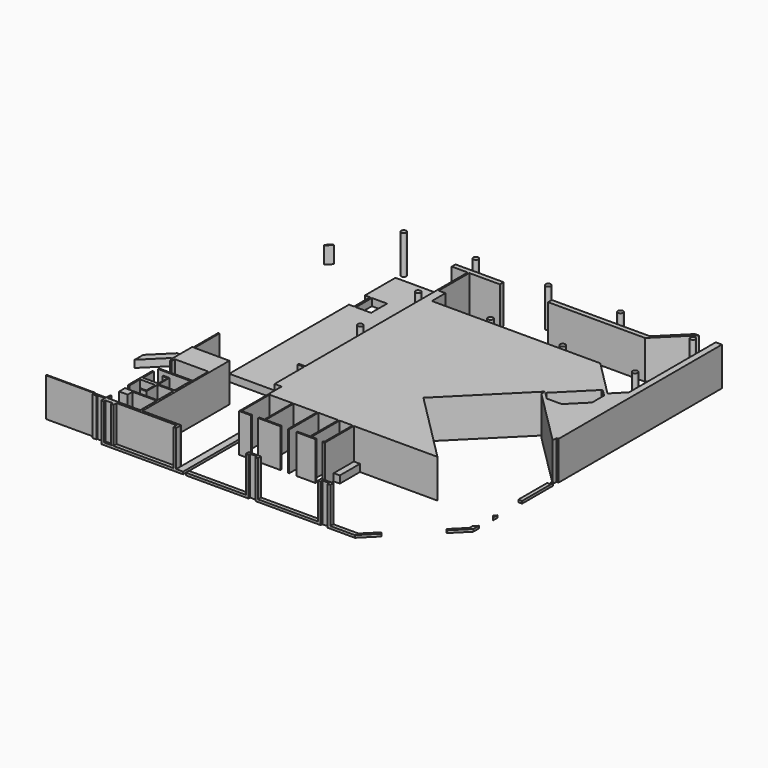
from build123d import *

# Parameters (mm, degrees)
F0_W      = 988.1219863892
F0_H      = 168.411863653
F1_DEPTH  = 4876.8
F0_R      = 328.452152689
F0_W_2    = 6102.4697852615
F0_H_2    = 118.2537078857
F2_DEPTH  = 914.4
F0_W_3    = 1924.9444007874
F0_H_3    = 2527.5359153748
F0_W_4    = 159.9474188251
F0_H_4    = 572.0329284668
F0_W_5    = 776.8564224243
F0_H_5    = 3188.3936524391
F3_DEPTH  = 177.8
F4_DEPTH  = 355.6
F5_DEPTH  = 533.4
F6_DEPTH  = 711.2
F7_DEPTH  = 889
F8_DEPTH  = 1066.8
F9_DEPTH  = 2133.6
F0_W_6    = 878.3769310551
F0_H_6    = 490.4985427856
F0_H_7    = 289.0536963655
F0_H_8    = 17331.1824798584
F0_H_9    = 184.3700408936
F0_H_10   = 7452.3627518665
F10_DEPTH = 304.8
F0_W_7    = 7604.6065750122
F0_W_8    = 7599.9544025821
F0_W_9    = 331.0794830322
F11_DEPTH = 4876.8


with BuildPart() as f1:
    # F0 (on Top) → F1 (new body)
    with BuildSketch(Plane.XY):
        Polygon((-9762.6952889996, -31763.6391877186), (-9950.2172235089, -31763.6391877186), (-9950.2172235089, -32382.503724004), (-9950.2172235089, -32550.915587657), (-9950.2172235089, -33159.8601280416), (-9619.1377404767, -33159.8601280416), (-9619.1377404767, -32907.453054067), (-8738.1992105084, -32907.453054067), (-8738.1992105084, -33145.5445228781), (-8410.8237985211, -33145.5445228781), (-8410.8237985211, -32669.361585256), (-806.2172235089, -32669.361585256), (-475.1377404767, -32669.361585256), (-475.1377404767, -32380.3078888905), (-5368.5698274213, -32380.3078888905), (-5368.5698274213, -18630.5877923023), (-9778.8629296857, -18630.5877923023), (-9778.8629296857, -15049.1254090321), (-9778.8629296857, -14864.7553681385), (-9778.8629296857, -14666.6457413685), (-9938.8103485107, -14666.6457413685), (-9938.8103485107, -15837.9578638238), (-9938.8103485107, -18630.5877923023), (-10073.0752944946, -18630.5877923023), (-10073.0752944946, -21932.6489324318), (-9941.6446450787, -21932.6489324318), (-9941.9820483797, -22319.5813578577), (-9762.6952889996, -22319.7376950899), (-9762.6952889996, -21738.5065316212), (-5534.9635842877, -21738.5065316212), (-5534.9635842877, -24228.4532546055), (-9762.6952889996, -24255.6560992252), (-9762.6952889996, -24422.071790601), (-5641.0493615704, -24422.071790601), (-5641.0493615704, -26945.4772233021), (-7697.0572236615, -26945.4772233021), (-7697.0572236615, -25199.2787479412), (-8474.8048782349, -25199.2787479412), (-8474.8048782349, -25341.5817229998), (-7804.6655419904, -25341.5817229998), (-7804.6655419904, -26805.3394316685), (-9762.6952889996, -26805.3394316685), (-9762.6952889996, -25341.5817229998), (-9762.6952889996, -25199.2787479412), (-9762.6952889996, -25087.7745624565), (-9944.395762002, -25087.6161204771), (-9947.7741608292, -28961.9470722609), (-9762.6952889996, -28961.9470722609), (-9762.6952889996, -28854.1154622089), (-9762.6952889996, -28712.3789547932), (-9762.6952889996, -27257.7159165394), (-7818.7813523846, -27257.7159165394), (-7818.7813523846, -28712.3789547932), (-8473.2656478882, -28712.3789547932), (-8473.2656478882, -28854.1154622089), (-7684.504962309, -28854.1154622089), (-7697.0572236615, -27101.0598896992), (-6705.3122520447, -27101.0598896992), (-5641.0493615704, -27101.0598896992), (-5641.0493615704, -27707.3329574996), (-5641.0493615704, -29643.5177086842), (-9762.6952889996, -29643.5177086842), (-9762.6952889996, -30572.3111390125), (-8683.9914086896, -30572.3111390125), (-8683.9914086896, -29799.5407341969), (-5641.0493615704, -29799.5407341969), (-5641.0493615704, -32380.3078888905), (-9762.6952889996, -32380.3078888905), align=None)
        Polygon((-10938.3392098981, -32550.915587657), (-10938.3392098981, -32382.503724004), (-11455.8429483014, -32382.503724004), (-11455.8429483014, -32680.3834198963), (-10938.3392098981, -32680.3834198963), align=None)
        with Locations((-10444.2782167035, -32466.7096558305)):
            Rectangle(F0_W, F0_H)
    extrude(amount=F1_DEPTH)

    # F0 (on Top) → F10 (join)
    with BuildSketch(Plane.XY):
        Polygon((-9619.1377404767, -32907.453054067), (-9619.1377404767, -33159.8601280416), (-806.2172235089, -33159.8601280416), (-806.2172235089, -32669.361585256), (-8410.8237985211, -32669.361585256), (-8410.8237985211, -33145.5445228781), (-8738.1992105084, -33145.5445228781), (-8738.1992105084, -32907.453054067), align=None)
        with Locations((-35.9492749491, -32914.6108566488)):
            Rectangle(F0_W_6, F0_H_6)
        with Locations((-35.9492749491, -32524.8347370732)):
            Rectangle(F0_W_6, F0_H_7)
        with Locations((-35.9492749491, -23714.7166489613)):
            Rectangle(F0_W_6, F0_H_8)
        with Locations((-35.9492749491, -14956.9403885853)):
            Rectangle(F0_W_6, F0_H_9)
        with Locations((-35.9492749491, -11138.5739922052)):
            Rectangle(F0_W_6, F0_H_10)
    extrude(amount=F10_DEPTH)


with BuildPart() as f1b:
    # F0 (on Top) → F1, piece 2 (new body)
    with BuildSketch(Plane.XY):
        Polygon((403.2391905785, -14864.7553681385), (403.2391905785, -15049.1254090321), (1221.1445804996, -15049.1254090321), (1221.1445804996, -19710.1065873158), (2114.7113081378, -19710.1065873158), (2114.7113081378, -20655.0921089583), (2114.7113081378, -20733.6380242359), (2114.7113081378, -26433.5496782314), (3611.5431785584, -26433.5496782314), (3611.5431785584, -26267.01645922), (2270.482301712, -26267.01645922), (2270.482301712, -21826.6788608962), (5186.9406700134, -21826.6788608962), (5186.9406700134, -26267.01645922), (4527.3551940918, -26267.01645922), (4527.3551940918, -26433.5496782314), (7342.5350189209, -26433.5496782314), (7342.5350189209, -26267.01645922), (5332.866191864, -26267.01645922), (5332.866191864, -21826.6788608962), (8282.6271057129, -21826.6788608962), (8282.6271057129, -26267.01645922), (8282.6271057129, -26433.5496782314), (8448.1201171875, -26433.5496782314), (8448.1201171875, -26267.01645922), (8448.1201171875, -21826.6788608962), (10967.3471450806, -21826.6788608962), (10967.3471450806, -26267.01645922), (9387.3443603516, -26267.01645922), (9387.3443603516, -26433.5496782314), (11770.4105377197, -26433.5496782314), (11770.4105377197, -26267.01645922), (11142.1804428101, -26267.01645922), (11142.1804428101, -21826.6788608962), (12795.4187393188, -21826.6788608962), (12795.4187393188, -26267.01645922), (12655.650138855, -26267.01645922), (12655.650138855, -26433.5496782314), (12953.9604422015, -26433.5496782314), (12953.9604422015, -25034.6246122372), (12953.9604422015, -21846.2309597981), (13730.8168646259, -21846.2309597981), (23534.5983740253, -21846.2309597981), (14549.2862374604, -12835.417128042), (23102.8533115337, -4306.0576854206), (23102.8533115337, -4877.016544342), (30215.8937689227, -11970.8853073243), (30215.8937689227, -11358.6764274801), (30472.748779909, -11358.6764274801), (30472.748779909, 14474.1640090942), (29691.0285949707, 14474.1640090942), (29691.0285949707, 751.9209384918), (28176.9048769071, -757.9176259485), (27421.1322496944, 0), (23591.3720324397, 3840.629664663), (2272.8099822998, 3840.629664663), (2272.8099822998, 5998.2261657715), (1416.9044729633, 5998.2261657715), (1416.9044729633, 10830.4662704468), (1221.1445804996, 10830.4662704468), (1221.1445804996, -14864.7553681385), align=None)
        with Locations((9121.6776853174, -4581.9952062592)):
            Circle(F0_R, mode=Mode.SUBTRACT)
        with Locations((18270.2025953174, -4581.9952062592)):
            Circle(F0_R, mode=Mode.SUBTRACT)
        Polygon((23372.4136352539, -4562.3035430908), (23372.4136352539, -4424.2610931396), (27250.2002716064, -545.2130857547), (27426.9443765413, -545.2130857547), (28200.6041700507, -1321.0686445236), (28200.6041700507, -2802.8049468994), (28200.6041700507, -3235.0963548069), (26065.6871795654, -5363.9712714722), (24176.2479287661, -5363.9712714722), align=None, mode=Mode.SUBTRACT)
        with Locations((9121.6776853174, -4581.9952062592)):
            Circle(F0_R)
        with Locations((18270.2025953174, -4581.9952062592)):
            Circle(F0_R)
        Polygon((-798.6393335896, 11424.7198104858), (-798.6393335896, 10830.4662704468), (1221.1445804996, 10830.4662704468), (1416.9044729633, 10830.4662704468), (5292.9373022479, 10830.4662704468), (5292.9373022479, 11424.7198104858), align=None)
    extrude(amount=F1_DEPTH)


with BuildPart() as f1c:
    # F0 (on Top) → F1, piece 3 (new body)
    with BuildSketch(Plane.XY):
        with Locations((-26.8472246826, 4554.5749137408)):
            Circle(F0_R)
    extrude(amount=F1_DEPTH)


with BuildPart() as f1d:
    # F0 (on Top) → F1, piece 4 (new body)
    with BuildSketch(Plane.XY):
        with Locations((-26.8472246826, -4581.9952062592)):
            Circle(F0_R)
    extrude(amount=F1_DEPTH)


with BuildPart() as f1e:
    # F0 (on Top) → F1, piece 5 (new body)
    with BuildSketch(Plane.XY):
        with Locations((-9163.0339622498, 13691.67878642)):
            Circle(F0_R)
    extrude(amount=F1_DEPTH)


with BuildPart() as f1f:
    # F0 (on Top) → F1, piece 6 (new body)
    with BuildSketch(Plane.XY):
        with Locations((-26.8472246826, 13691.1450337408)):
            Circle(F0_R)
    extrude(amount=F1_DEPTH)


with BuildPart() as f1g:
    # F0 (on Top) → F1, piece 7 (new body)
    with BuildSketch(Plane.XY):
        with Locations((9121.6776853174, 4554.5749137408)):
            Circle(F0_R)
    extrude(amount=F1_DEPTH)


with BuildPart() as f1h:
    # F0 (on Top) → F1, piece 8 (new body)
    with BuildSketch(Plane.XY):
        with Locations((9121.6776853174, 13691.1450337408)):
            Circle(F0_R)
    extrude(amount=F1_DEPTH)


with BuildPart() as f1i:
    # F0 (on Top) → F1, piece 9 (new body)
    with BuildSketch(Plane.XY):
        with Locations((18270.2025953174, 13691.1450337408)):
            Circle(F0_R)
    extrude(amount=F1_DEPTH)


with BuildPart() as f1j:
    # F0 (on Top) → F1, piece 10 (new body)
    with BuildSketch(Plane.XY):
        with Locations((18270.2025953174, 4554.5749137408)):
            Circle(F0_R)
    extrude(amount=F1_DEPTH)


with BuildPart() as f1k:
    # F0 (on Top) → F1, piece 11 (new body)
    with BuildSketch(Plane.XY):
        with Locations((27432.5160980225, 4548.7937927246)):
            Circle(F0_R)
    extrude(amount=F1_DEPTH)


with BuildPart() as f1l:
    # F0 (on Top) → F1, piece 12 (new body)
    with BuildSketch(Plane.XY):
        with Locations((27415.8744812012, 13708.9691162109)):
            Circle(F0_R)
    extrude(amount=F1_DEPTH)


with BuildPart() as f1m:
    # F0 (on Top) → F1, piece 13 (new body)
    with BuildSketch(Plane.XY):
        with Locations((-14507.0778409321, -32323.3768700611)):
            Rectangle(F0_W_2, F0_H_2)
    extrude(amount=F1_DEPTH)


with BuildPart() as f1n:
    # F0 (on Top) → F1, piece 14 (new body)
    with BuildSketch(Plane.XY):
        Polygon((23506.2954206457, 11424.7198104858), (11396.935486452, 11424.7198104858), (11396.935486452, 10830.4662704468), (23674.6969458026, 10830.4662704468), (27462.4419350844, 14581.0467946258), (26998.763107912, 14581.0467946258), (23811.1601110858, 11424.7198104858), (23591.9761657715, 11424.7198104858), align=None)
    extrude(amount=F1_DEPTH)

    # F0 (on Top) → F3 (join)
    with BuildSketch(Plane.XY):
        Polygon((20380.9375762939, 14581.0467946258), (23506.2954206457, 11424.7198104858), (23591.9761657715, 11424.7198104858), (23773.1500730023, 11604.1160818484), (23772.2745090816, 11605.0003217233), (20825.4283058909, 14581.0467946258), align=None)
    extrude(amount=F3_DEPTH)

    # F0 (on Top) → F4 (join)
    with BuildSketch(Plane.XY):
        Polygon((21236.7263575649, 14581.0467946258), (20825.4283058909, 14581.0467946258), (23772.2745090816, 11605.0003217233), (23979.9512134187, 11810.6393509654), (23977.6984338147, 11812.91445334), align=None)
    extrude(amount=F4_DEPTH)

    # F0 (on Top) → F5 (join)
    with BuildSketch(Plane.XY):
        Polygon((21619.1883087158, 14581.0467946258), (21236.7263575649, 14581.0467946258), (23977.6984338147, 11812.91445334), (24170.8149273796, 12004.1361331816), align=None)
    extrude(amount=F5_DEPTH)

    # F0 (on Top) → F6 (join)
    with BuildSketch(Plane.XY):
        Polygon((22054.3809336063, 14581.0467946258), (21619.1883087158, 14581.0467946258), (24170.8149273796, 12004.1361331816), (24390.556717357, 12221.7218682746), align=None)
    extrude(amount=F6_DEPTH)

    # F0 (on Top) → F7 (join)
    with BuildSketch(Plane.XY):
        Polygon((22442.3141479492, 14581.0467946258), (22054.3809336063, 14581.0467946258), (24390.556717357, 12221.7218682746), (24593.3447991154, 12422.5202409557), align=None)
    extrude(amount=F7_DEPTH)

    # F0 (on Top) → F8 (join)
    with BuildSketch(Plane.XY):
        Polygon((26759.3933769787, 14581.0467946258), (22442.3141479492, 14581.0467946258), (24593.3447991154, 12422.5202409557), align=None)
    extrude(amount=F8_DEPTH)


with BuildPart() as f2:
    # F0 (on Top) → F2 (new body)
    with BuildSketch(Plane.XY):
        Polygon((-14995.7607054516, -15837.9578638238), (-10073.0752944946, -15837.9578638238), (-10073.0752944946, -14666.6457413685), (-11468.9082864362, -14666.6457413685), (-11468.9082864362, -14647.9565857899), (-15154.6497109967, -14647.9565857899), (-17558.3127335629, -17028.1916874721), (-17558.3127335629, -18375.5333184254), align=None)
    extrude(amount=F2_DEPTH)


with BuildPart() as f2b:
    # F0 (on Top) → F2, piece 2 (new body)
    with BuildSketch(Plane.XY):
        Polygon((-8397.25110565, -14864.7553681385), (-798.6393335896, -14864.7553681385), (-798.6393335896, 10830.4662704468), (-798.6393335896, 11424.7198104858), (-8397.25110565, 11424.7198104858), (-8397.25110565, 6600.5563735962), (-7756.338596344, 6600.5563735962), (-7756.338596344, 4073.0204582214), (-8397.25110565, 4073.0204582214), (-8397.25110565, -14075.9236573231), (-8397.25110565, -14666.6457413685), align=None)
        with Locations((-6551.1560440063, 5328.4192085266)):
            Rectangle(F0_W_3, F0_H_3, mode=Mode.SUBTRACT)
    extrude(amount=F2_DEPTH)


with BuildPart() as f2c:
    # F0 (on Top) → F2, piece 3 (new body)
    with BuildSketch(Plane.XY):
        with Locations((-9858.8366390982, -14361.9401215565)):
            Rectangle(F0_W_4, F0_H_4)
    extrude(amount=F2_DEPTH)


with BuildPart() as f2d:
    # F0 (on Top) → F2, piece 4 (new body)
    with BuildSketch(Plane.XY):
        with Locations((13342.3886534137, -23440.4277860176)):
            Rectangle(F0_W_5, F0_H_5)
    extrude(amount=F2_DEPTH)


with BuildPart() as f9:
    # F0 (on Top) → F9 (new body)
    with BuildSketch(Plane.XY):
        Polygon((-16165.1107208616, 11354.981127925), (-16854.9365997314, 10671.8788146973), (-16764.5554840304, 10580.6081055159), (-16074.7296051605, 11263.7104187436), align=None)
    extrude(amount=F9_DEPTH)


with BuildPart() as f10:
    # F0 (on Top) → F10, piece 2 (new body)
    with BuildSketch(Plane.XY):
        with Locations((13679.479488985, -32914.6108566488)):
            Rectangle(F0_W_7, F0_H_6)
    extrude(amount=F10_DEPTH)


with BuildPart() as f10b:
    # F0 (on Top) → F10, piece 3 (new body)
    with BuildSketch(Plane.XY):
        Polygon((22197.7644201678, -32669.361585256), (19021.1762014789, -32669.361585256), (19021.1762014789, -33159.8601280416), (22137.6570497929, -33159.8601280416), (24012.823326375, -31290.0007992792), (23797.5435491962, -31074.1100250448), align=None)
    extrude(amount=F10_DEPTH)


with BuildPart() as f10c:
    # F0 (on Top) → F10, piece 4 (new body)
    with BuildSketch(Plane.XY):
        Polygon((30471.1427923602, -21395.8024917806), (30471.1427923602, -21715.7225547994), (30471.2464549473, -21047.2004379609), (30212.2297521991, -21305.4840920493), (30212.2297521991, -21395.8024917806), align=None)
    extrude(amount=F10_DEPTH)


with BuildPart() as f10d:
    # F0 (on Top) → F10, piece 5 (new body)
    with BuildSketch(Plane.XY):
        Polygon((30471.8532292104, -17134.1009640984), (30472.6141490196, -12226.9137519957), (30215.8937689227, -11970.8853073243), (30215.8937689227, -12236.5841804708), (30453.5745818257, -12236.5841804708), (30453.5745818257, -12570.6650188443), (30000.2853813181, -12570.1126991476), (29994.7250028424, -17133.5195972426), align=None)
    extrude(amount=F10_DEPTH)


with BuildPart() as f10e:
    # F0 (on Top) → F10, piece 6 (new body)
    with BuildSketch(Plane.XY):
        Polygon((30466.0057710437, -23927.4486224129), (30000.2853813182, -24394.4276552413), (30000.2853813181, -24882.9862926356), (28388.3199833464, -26490.3896331723), (28592.1354528827, -26694.7835622991), (30463.9134197477, -24828.3029539267), align=None)
    extrude(amount=F10_DEPTH)


with BuildPart() as f10f:
    # F0 (on Top) → F10, piece 7 (new body)
    with BuildSketch(Plane.XY):
        with Locations((4537.8055752, -32914.6108566488)):
            Rectangle(F0_W_8, F0_H_6)
    extrude(amount=F10_DEPTH)


with BuildPart() as f11:
    # F0 (on Top) → F11 (new body)
    with BuildSketch(Plane.XY):
        with Locations((-640.6774819928, -32914.6108566488)):
            Rectangle(F0_W_9, F0_H_6)
    extrude(amount=F11_DEPTH)


with BuildPart() as f11b:
    # F0 (on Top) → F11, piece 2 (new body)
    with BuildSketch(Plane.XY):
        Polygon((8337.7827764911, -32669.361585256), (8337.7827764911, -33159.8601280416), (8668.8622595233, -33159.8601280416), (8668.8622595233, -32907.453054067), (9549.8007894916, -32907.453054067), (9549.8007894916, -33159.8601280416), (9877.1762014789, -33159.8601280416), (9877.1762014789, -32669.361585256), align=None)
    extrude(amount=F11_DEPTH)


with BuildPart() as f11c:
    # F0 (on Top) → F11, piece 3 (new body)
    with BuildSketch(Plane.XY):
        Polygon((19021.1762014789, -32669.361585256), (17481.7827764911, -32669.361585256), (17481.7827764911, -33159.8601280416), (17812.8622595233, -33159.8601280416), (17816.7476654053, -33159.8601280416), (17812.8622595233, -32907.453054067), (18693.8007894916, -32907.453054067), (18693.8007894916, -33145.5445228781), (18693.8007894916, -33159.8601280416), (19021.1762014789, -33159.8601280416), align=None)
    extrude(amount=F11_DEPTH)


solid = Compound([f1.part, f1b.part, f1c.part, f1d.part, f1e.part, f1f.part, f1g.part, f1h.part, f1i.part, f1j.part, f1k.part, f1l.part, f1m.part, f1n.part, f2.part, f2b.part, f2c.part, f2d.part, f9.part, f10.part, f10b.part, f10c.part, f10d.part, f10e.part, f10f.part, f11.part, f11b.part, f11c.part])
